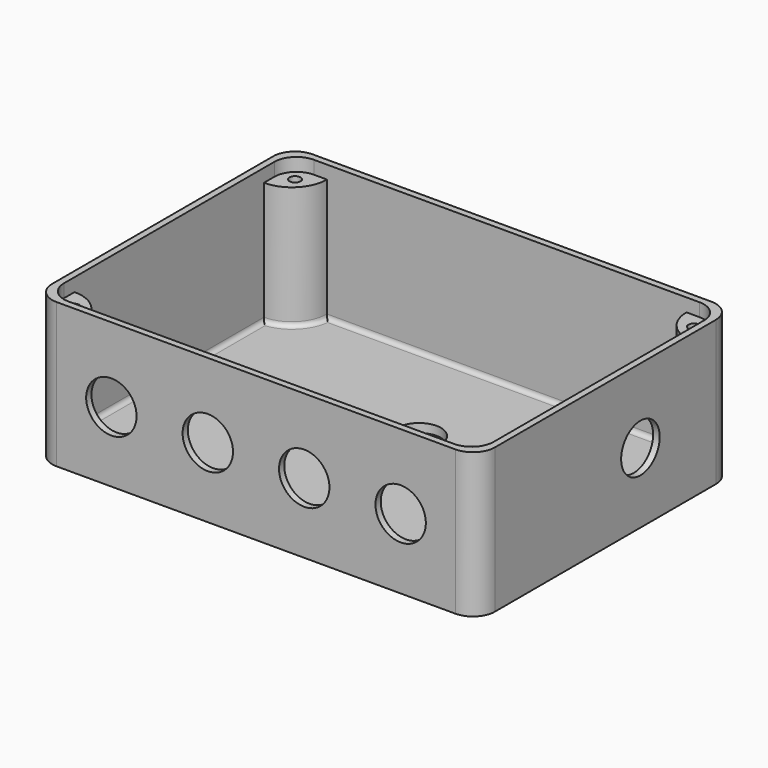
from build123d import *

# Parameters (mm, degrees)
F0_R      = 1.25
F1_DEPTH  = 2
F0_W      = 101
F0_H      = 73
F2_DEPTH  = 30
F3_DEPTH  = 33
F4_R      = 5.5
F5_DEPTH  = 2
F6_R      = 5.75
F7_DEPTH  = 2
F8_R      = 1
F9_R      = 5
F10_R     = 5
F10_R_2   = 1.8
F11_DEPTH = 5


# Not quite as in the source:
# - a feature names something its author has since deleted; it is built from what else it names


with BuildPart() as f1:
    # F0 (on Top) → F1 (new body)
    with BuildSketch(Plane.XY):
        with BuildLine():
            Line((41, -45), (49, -45))
            Line((49, -45), (49, -37))
            ThreePointArc((49, -37), (43.3431457505, -39.3431457505), (41, -45))
        make_face()
        with Locations((45.5, -41.5)):
            Circle(F0_R, mode=Mode.SUBTRACT)
        with BuildLine():
            Line((-41, -45), (41, -45))
            ThreePointArc((41, -45), (43.3431457505, -39.3431457505), (49, -37))
            Line((49, -37), (49, 17))
            ThreePointArc((49, 17), (43.3431457505, 19.3431457505), (41, 25))
            Line((41, 25), (-41, 25))
            ThreePointArc((-41, 25), (-43.3431457505, 19.3431457505), (-49, 17))
            Line((-49, 17), (-49, -37))
            ThreePointArc((-49, -37), (-43.3431457505, -39.3431457505), (-41, -45))
        make_face()
        with BuildLine():
            Line((-49, -45), (-41, -45))
            ThreePointArc((-41, -45), (-43.3431457505, -39.3431457505), (-49, -37))
            Line((-49, -37), (-49, -45))
        make_face()
        with Locations((-45.5, -41.5)):
            Circle(F0_R, mode=Mode.SUBTRACT)
        with BuildLine():
            Line((-49, 25), (-49, 17))
            ThreePointArc((-49, 17), (-43.3431457505, 19.3431457505), (-41, 25))
            Line((-41, 25), (-49, 25))
        make_face()
        with Locations((-45.5, 21.5)):
            Circle(F0_R, mode=Mode.SUBTRACT)
        with Locations((-45.5, 21.5)):
            Circle(F0_R)
        with BuildLine():
            ThreePointArc((41, 25), (43.3431457505, 19.3431457505), (49, 17))
            Line((49, 17), (49, 25))
            Line((49, 25), (41, 25))
        make_face()
        with Locations((45.5, 21.5)):
            Circle(F0_R, mode=Mode.SUBTRACT)
        with Locations((45.5, 21.5)):
            Circle(F0_R)
        with Locations((45.5, -41.5)):
            Circle(F0_R)
        with Locations((-45.5, -41.5)):
            Circle(F0_R)
    extrude(amount=F1_DEPTH)

    # F0 (on Top) → F2 (join)
    with BuildSketch(Plane.XY):
        with Locations((0, -10)):
            Rectangle(F0_W, F0_H)
        Polygon((49, -37), (49, -45), (41, -45), (-41, -45), (-49, -45), (-49, -37), (-49, 17), (-49, 25), (-41, 25), (41, 25), (49, 25), (49, 17), align=None, mode=Mode.SUBTRACT)
        with BuildLine():
            Line((-49, -45), (-41, -45))
            ThreePointArc((-41, -45), (-43.3431457505, -39.3431457505), (-49, -37))
            Line((-49, -37), (-49, -45))
        make_face()
        with Locations((-45.5, -41.5)):
            Circle(F0_R, mode=Mode.SUBTRACT)
        with BuildLine():
            Line((41, -45), (49, -45))
            Line((49, -45), (49, -37))
            ThreePointArc((49, -37), (43.3431457505, -39.3431457505), (41, -45))
        make_face()
        with Locations((45.5, -41.5)):
            Circle(F0_R, mode=Mode.SUBTRACT)
        with BuildLine():
            ThreePointArc((41, 25), (43.3431457505, 19.3431457505), (49, 17))
            Line((49, 17), (49, 25))
            Line((49, 25), (41, 25))
        make_face()
        with Locations((45.5, 21.5)):
            Circle(F0_R, mode=Mode.SUBTRACT)
        with BuildLine():
            Line((-49, 25), (-49, 17))
            ThreePointArc((-49, 17), (-43.3431457505, 19.3431457505), (-41, 25))
            Line((-41, 25), (-49, 25))
        make_face()
        with Locations((-45.5, 21.5)):
            Circle(F0_R, mode=Mode.SUBTRACT)
    extrude(amount=F2_DEPTH)

    # F0 (on Top) → F3 (join)
    with BuildSketch(Plane.XY):
        with Locations((0, -10)):
            Rectangle(F0_W, F0_H)
        Polygon((49, -37), (49, -45), (41, -45), (-41, -45), (-49, -45), (-49, -37), (-49, 17), (-49, 25), (-41, 25), (41, 25), (49, 25), (49, 17), align=None, mode=Mode.SUBTRACT)
    extrude(amount=F3_DEPTH)

    # F4 (on face) → F5 (cut)
    with BuildSketch(Plane.YZ.offset(50.5)):
        with Locations((0, 16)):
            Circle(F4_R)
    extrude(amount=-F5_DEPTH, mode=Mode.SUBTRACT)

    # F6 (on face) → F7 (cut)
    with BuildSketch(Plane.XZ.offset(46.5)):
        with Locations((-33, 16)):
            Circle(F6_R)
        with Locations((-11, 16)):
            Circle(F6_R)
        with Locations((11, 16)):
            Circle(F6_R)
        with Locations((33, 16)):
            Circle(F6_R)
    extrude(amount=-F7_DEPTH, mode=Mode.SUBTRACT)

    # F8
    f8_edges = [f1.edges().sort_by_distance(p)[0] for p in [
        (0, -45, 2),
        (-49, -10, 2),
        (0, 25, 2),
        (49, -10, 2),
        (43.343146, -39.343146, 2),
        (43.343146, 19.343146, 2),
        (-43.343146, 19.343146, 2),
        (-43.343146, -39.343146, 2),
    ]]
    fillet(f8_edges, radius=F8_R)

    # F9
    f9_edges = [f1.edges().sort_by_distance(p)[0] for p in [
        (-50.5, 26.5, 16.5),
        (50.5, 26.5, 16.5),
        (50.5, -46.5, 16.5),
        (-50.5, -46.5, 16.5),
        (49, -45, 31.5),
        (49, 25, 31.5),
        (-49, 25, 31.5),
        (-49, -45, 31.5),
    ]]
    fillet(f9_edges, radius=F9_R)

    # F10 (on face) → F11 (cut)
    with BuildSketch(Plane(origin=(0, 0, 0), x_dir=(1, 0, 0), z_dir=(0, 0, -1))):
        Circle(F10_R)
        with Locations((0, 9.5)):
            Circle(F10_R_2)
    extrude(amount=-F11_DEPTH, mode=Mode.SUBTRACT)


solid = f1.part
